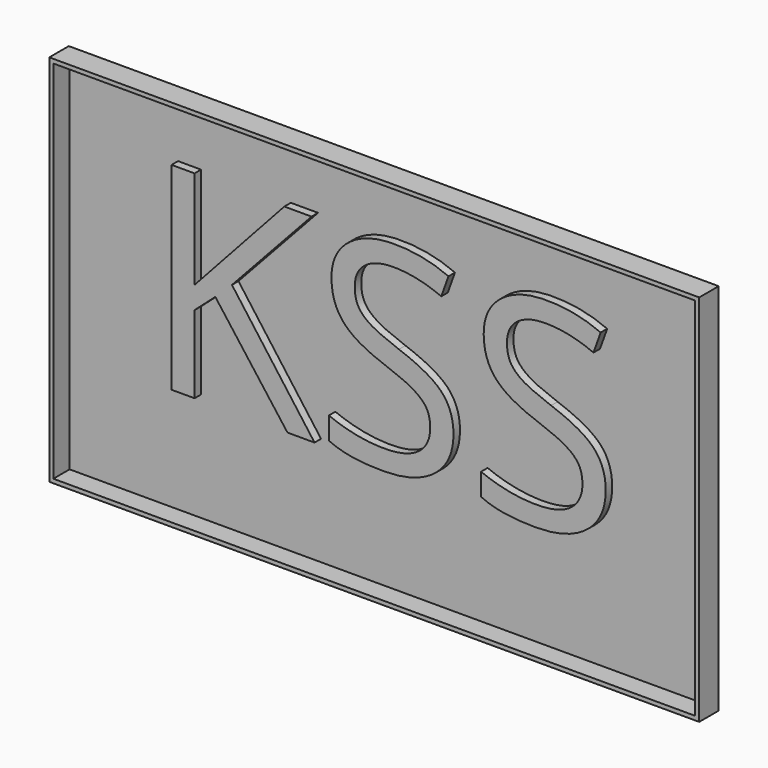
from build123d import *

# Parameters (mm, degrees)
F0_W         = 400
F0_H         = 230
F1_DEPTH     = 15
F2_T         = -2.5
F3_R         = 15
F4_DEPTH     = 0.5
F5_TEXT_SIZE = 170.674380763
F6_DEPTH     = 5


# Not quite as in the source:
# - Text() gives the source's letters only with a copy of the font that has no kerning and outlines rounded to 1/6400 em; it was checked with that copy


with BuildPart() as f1:
    # F0 (on Front) → F1 (new body)
    with BuildSketch(Plane.XZ):
        Rectangle(F0_W, F0_H)
    extrude(amount=F1_DEPTH)

    # F2
    f2_openings = [f1.faces().sort_by_distance(p)[0] for p in [
        (0, -15, 0),
    ]]
    offset(amount=F2_T, openings=f2_openings)

    # F3 (on face) → F4 (cut)
    with BuildSketch(Plane(origin=(0, 0, 0), x_dir=(-1, 0, 0), z_dir=(0, 1, 0))):
        Circle(F3_R)
    extrude(amount=-F4_DEPTH, mode=Mode.SUBTRACT)

    # F5 (on face) → F6 (join)
    with BuildSketch(Plane.XZ.offset(2.5)):
        with Locations((-147.5, -45.6409981296)):
            Text('KSS', F5_TEXT_SIZE, font='Open Sans', text_align=(TextAlign.LEFT, TextAlign.BOTTOM))
    extrude(amount=F6_DEPTH)


solid = f1.part
